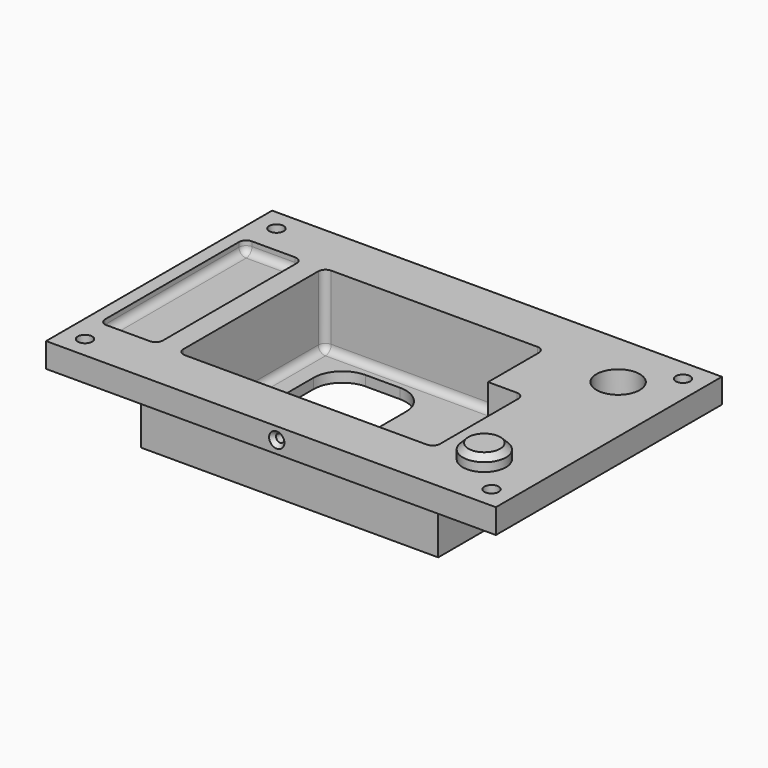
from build123d import *

# Parameters (mm, degrees)
F0_W            = 396.24
F0_H            = 248.92
F1_DEPTH        = 21.59
F3_DEPTH        = 50.8
F5_DEPTH        = 63.5
F6_R            = 6.35
F7_R            = 5.08
F8_W            = 81.28
F8_H            = 137.16
F9_DEPTH        = 72.391
F10_W           = 50.8
F10_H           = 160.02
F11_DEPTH       = 10.414
F12_R           = 6.35
F13_R           = 19.05
F14_DEPTH       = 12.7
F15_SIZE        = 5.08
F17_D           = 7.1374
F17_DEPTH       = 127
F17_CSINK_D     = 13.4874
F17_CSINK_ANGLE = 82
F17_TIP         = 2.1442912911
F19_D           = 12.7
F19_CBORE_D     = 22.225
F19_CBORE_DEPTH = 12.7
F20_R           = 19.05
F21_DEPTH       = 72.391
F22_R           = 25.4


with BuildPart() as f1:
    # F0 (on Top) → F1 (new body)
    with BuildSketch(Plane.XY):
        Rectangle(F0_W, F0_H)
    extrude(amount=-F1_DEPTH)

    # F2 (on face) → F3 (join)
    with BuildSketch(Plane(origin=(0, 0, -21.59), x_dir=(1, 0, 0), z_dir=(0, 0, -1))):
        Polygon((127, 99.06), (-134.62, 99.06), (-134.62, -97.79), (95.25, -97.79), (95.25, -35.56), (127, -35.56), align=None)
    extrude(amount=F3_DEPTH)

    # F4 (on face) → F5 (cut)
    with BuildSketch(Plane.XY):
        Polygon((-116.84, -81.28), (109.22, -81.28), (109.22, 17.78), (77.47, 17.78), (77.47, 80.01), (-116.84, 80.01), align=None)
    extrude(amount=-F5_DEPTH, mode=Mode.SUBTRACT)

    # F6
    f6_edges = [f1.edges().sort_by_distance(p)[0] for p in [
        (-3.81, -81.28, -63.5),
        (109.22, -31.75, -63.5),
        (93.345, 17.78, -63.5),
        (77.47, 48.895, -63.5),
        (-19.685, 80.01, -63.5),
        (-116.84, -0.635, -63.5),
        (109.22, -81.28, -31.75),
        (-116.84, -81.28, -31.75),
        (-116.84, 80.01, -31.75),
        (109.22, 17.78, -31.75),
        (77.47, 80.01, -31.75),
    ]]
    fillet(f6_edges, radius=F6_R)

    # F7
    f7_edges = [f1.edges().sort_by_distance(p)[0] for p in [
        (95.25, 35.56, -46.99),
    ]]
    fillet(f7_edges, radius=F7_R)

    # F8 (on face) → F9 (cut, through all)
    with BuildSketch(Plane(origin=(0, 0, -72.39), x_dir=(1, 0, 0), z_dir=(0, 0, -1))):
        with Locations((-55.88, 0)):
            Rectangle(F8_W, F8_H)
    extrude(amount=-F9_DEPTH, mode=Mode.SUBTRACT)

    # F10 (on face) → F11 (cut)
    with BuildSketch(Plane.XY):
        with Locations((-161.29, 0)):
            Rectangle(F10_W, F10_H)
    extrude(amount=-F11_DEPTH, mode=Mode.SUBTRACT)

    # F12
    f12_edges = [f1.edges().sort_by_distance(p)[0] for p in [
        (-135.89, 0, -10.414),
        (-161.29, 80.01, -10.414),
        (-186.69, 0, -10.414),
        (-161.29, -80.01, -10.414),
        (-186.69, 80.01, -5.207),
        (-135.89, 80.01, -5.207),
        (-135.89, -80.01, -5.207),
        (-186.69, -80.01, -5.207),
    ]]
    fillet(f12_edges, radius=F12_R)

    # F13 (on face) → F14 (join)
    with BuildSketch(Plane.XY):
        with Locations((147.32, -73.66)):
            Circle(F13_R)
    extrude(amount=F14_DEPTH)

    # F15
    f15_edges = [f1.edges().sort_by_distance(p)[0] for p in [
        (128.27, -73.66, 12.7),
    ]]
    chamfer(f15_edges, length=F15_SIZE)

    # F17
    with Locations(Plane.XZ.offset(124.46)):
        with Locations((5.08, -10.668)):
            CounterSinkHole(F17_D / 2, F17_CSINK_D / 2, depth=F17_DEPTH, counter_sink_angle=F17_CSINK_ANGLE)
            with Locations((0, 0, -(F17_DEPTH + F17_TIP / 2))):  # 118° drill point
                Cone(0, F17_D / 2, F17_TIP, mode=Mode.SUBTRACT)

    # F19 (through all)
    with Locations(Plane(origin=(0, 0, -21.59), x_dir=(1, 0, 0), z_dir=(0, 0, -1))):
        with Locations((-179.07, 105.41), (179.07, 105.41), (179.07, -105.41), (-179.07, -105.41)):
            CounterBoreHole(F19_D / 2, F19_CBORE_D / 2, F19_CBORE_DEPTH)

    # F20 (on face) → F21 (cut, through all)
    with BuildSketch(Plane.XY):
        with Locations((147.32, 73.66)):
            Circle(F20_R)
    extrude(amount=-F21_DEPTH, mode=Mode.SUBTRACT)

    # F22
    f22_edges = [f1.edges().sort_by_distance(p)[0] for p in [
        (-15.24, -68.58, -67.945),
        (-15.24, 68.58, -67.945),
        (-96.52, 68.58, -67.945),
        (-96.52, -68.58, -67.945),
    ]]
    fillet(f22_edges, radius=F22_R)


solid = f1.part
